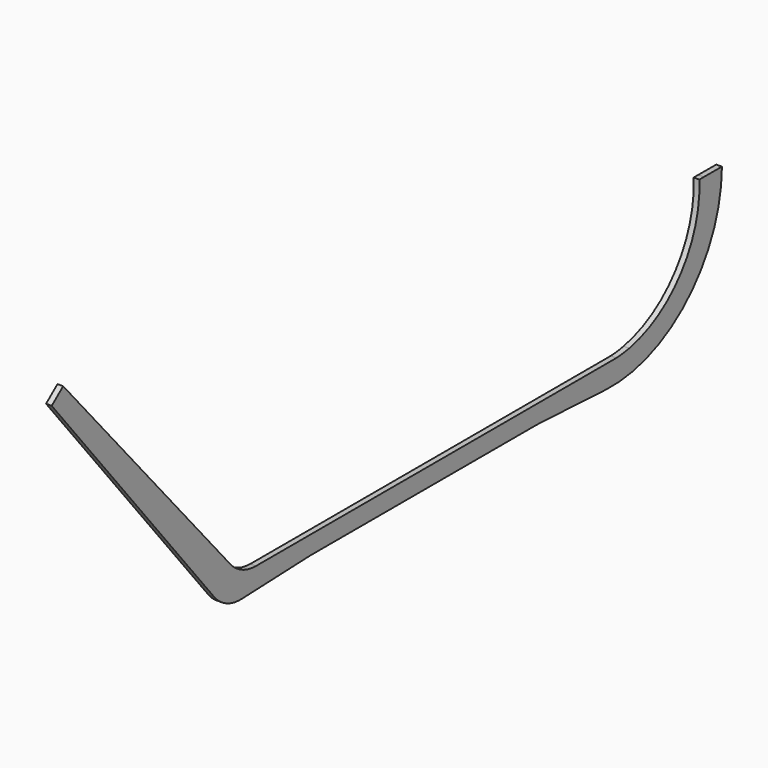
from build123d import *

# Parameters (mm, degrees)
F1_DEPTH = 4


# Not quite as in the source:
# - a feature names something its author has since deleted; it is built from what else it names


with BuildPart() as f1:
    # F0 (on Right) → F1 (new body)
    with BuildSketch(Plane.YZ):
        with BuildLine():
            Line((-151.036893852, 186.5150307497), (-7.0347090015, 8.6871421429))
            ThreePointArc((-7.0347090015, 8.6871421429), (4.1862889829, 0.1122435093), (18.0871758973, -2.3787453176))
            Line((18.0871758973, -2.3787453176), (76.0584955576, -0.0786202013))
            ThreePointArc((76.0584955576, -0.0786202013), (78.0403935877, -0.0196569823), (80.023071087, 0))
            Line((80.023071087, 0), (275.0031210998, 0))
            ThreePointArc((275.0031210998, 0), (279.998441154, -0.0623927883), (284.9906444886, -0.2495322244))
            Line((284.9906444886, -0.2495322244), (340, -3))
            ThreePointArc((340, -3), (412.2291799256, 23.705892636), (442.8144690376, 94.379786148))
            Line((442.8144690376, 94.379786148), (426.8144690376, 94.448943804))
            Line((426.8144690376, 94.448943804), (422.8144690376, 94.448943804))
            ThreePointArc((422.8144690376, 94.448943804), (406.6400435708, 42.8631388402), (360.6700266042, 14.4120430259))
            ThreePointArc((360.6700266042, 14.4120430259), (355.0395932087, 13.5090940512), (349.3599875605, 13))
            Line((349.3599875605, 13), (29.918677403, 13))
            ThreePointArc((29.918677403, 13), (17.4430940609, 15.7170415777), (7.2272892953, 23.3760119817))
            Line((7.2272892953, 23.3760119817), (-140.933996353, 194.6961958333))
            Line((-140.933996353, 194.6961958333), (-151.036893852, 186.5150307497))
        make_face()
    extrude(amount=F1_DEPTH)


solid = f1.part
